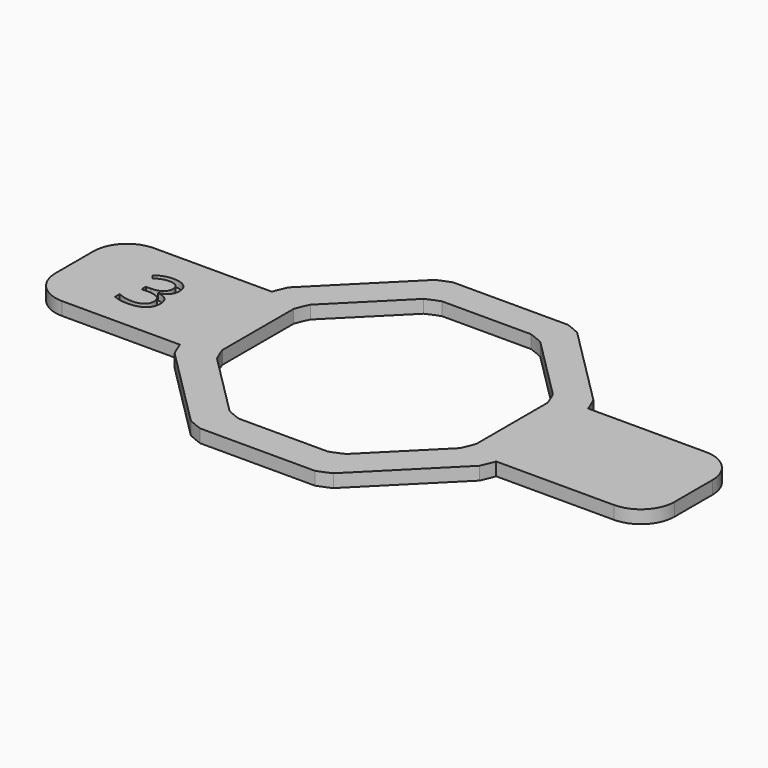
from build123d import *

# Parameters (mm, degrees)
F1_DEPTH     = 1.27
F2_DEPTH     = 1.27
F0_TEXT_SIZE = 7.2862855935
F3_DEPTH     = 0.635


# Not quite as in the source:
# - Text() gives the source's letters only with a copy of the font that has no kerning and outlines rounded to 1/6400 em; it was checked with that copy


with BuildPart() as f1:
    # F0 (on Top) → F1 (new body)
    with BuildSketch(Plane.XY):
        with BuildLine():
            Line((-6.9140659899, 14.7924959485), (-14.7924959485, 6.9140659899))
            ThreePointArc((-14.7924959485, 6.9140659899), (-15.085632938, 6.2486737599), (-15.3488571429, 5.5708912488))
            Line((-15.3488571429, 5.5708912488), (-15.3488571429, -5.5708912488))
            ThreePointArc((-15.3488571429, -5.5708912488), (-15.085632938, -6.2486737599), (-14.7924959485, -6.9140659899))
            Line((-14.7924959485, -6.9140659899), (-6.9140659899, -14.7924959485))
            ThreePointArc((-6.9140659899, -14.7924959485), (-6.2486737599, -15.085632938), (-5.5708912488, -15.3488571429))
            Line((-5.5708912488, -15.3488571429), (5.5708912488, -15.3488571429))
            ThreePointArc((5.5708912488, -15.3488571429), (6.2486737599, -15.085632938), (6.9140659899, -14.7924959485))
            Line((6.9140659899, -14.7924959485), (14.7924959485, -6.9140659899))
            ThreePointArc((14.7924959485, -6.9140659899), (15.085632938, -6.2486737599), (15.3488571429, -5.5708912488))
            Line((15.3488571429, -5.5708912488), (15.3488571429, 5.5708912488))
            ThreePointArc((15.3488571429, 5.5708912488), (15.085632938, 6.2486737599), (14.7924959485, 6.9140659899))
            Line((14.7924959485, 6.9140659899), (6.9140659899, 14.7924959485))
            ThreePointArc((6.9140659899, 14.7924959485), (6.2486737599, 15.085632938), (5.5708912488, 15.3488571429))
            Line((5.5708912488, 15.3488571429), (-5.5708912488, 15.3488571429))
            ThreePointArc((-5.5708912488, 15.3488571429), (-6.2486737599, 15.085632938), (-6.9140659899, 14.7924959485))
        make_face()
        with BuildLine():
            ThreePointArc((11.8104123626, 5.726089617), (12.1074053598, 5.0620161659), (12.366970438, 4.3824395631))
            Line((12.366970438, 4.3824395631), (12.366970438, -4.2562852471))
            ThreePointArc((12.366970438, -4.2562852471), (12.1074053598, -4.9358618499), (11.8104123626, -5.599935301))
            Line((11.8104123626, -5.599935301), (5.7019114684, -11.7084361952))
            ThreePointArc((5.7019114684, -11.7084361952), (5.0378380173, -12.0054291924), (4.3582614145, -12.2649942706))
            Line((4.3582614145, -12.2649942706), (-4.2804633957, -12.2649942706))
            ThreePointArc((-4.2804633957, -12.2649942706), (-4.9600399985, -12.0054291924), (-5.6241134496, -11.7084361952))
            Line((-5.6241134496, -11.7084361952), (-11.7326143438, -5.599935301))
            ThreePointArc((-11.7326143438, -5.599935301), (-12.029607341, -4.9358618499), (-12.2891724192, -4.2562852471))
            Line((-12.2891724192, -4.2562852471), (-12.2891724192, 4.3824395631))
            ThreePointArc((-12.2891724192, 4.3824395631), (-12.029607341, 5.0620161659), (-11.7326143438, 5.726089617))
            Line((-11.7326143438, 5.726089617), (-5.6241134496, 11.8345905111))
            ThreePointArc((-5.6241134496, 11.8345905111), (-4.9600399985, 12.1315835084), (-4.2804633957, 12.3911485866))
            Line((-4.2804633957, 12.3911485866), (4.3582614145, 12.3911485866))
            ThreePointArc((4.3582614145, 12.3911485866), (5.0378380173, 12.1315835084), (5.7019114684, 11.8345905111))
            Line((5.7019114684, 11.8345905111), (11.8104123626, 5.726089617))
        make_face(mode=Mode.SUBTRACT)
    extrude(amount=F1_DEPTH)

    # F0 (on Top) → F2 (join)
    with BuildSketch(Plane.XY):
        with BuildLine():
            Line((-15.3488571429, -5.5708912488), (-15.3488571429, 5.5708912488))
            Line((-15.3488571429, 5.5708912488), (-26.7788571429, 5.5708912488))
            ThreePointArc((-26.7788571429, 5.5708912488), (-29.0880658597, 4.6143856799), (-30.0445714286, 2.3051769631))
            Line((-30.0445714286, 2.3051769631), (-30.0445714286, -2.3051769631))
            ThreePointArc((-30.0445714286, -2.3051769631), (-29.0880658597, -4.6143856799), (-26.7788571429, -5.5708912488))
            Line((-26.7788571429, -5.5708912488), (-15.3488571429, -5.5708912488))
        make_face()
        with BuildLine():
            add(Edge.make_bspline(
                [(-21.2788977233, 2.223162781), (-20.8587978195, 1.8764949743), (-20.8587978195, 1.2719609664)],
                knots=[0, 0, 0, 1, 1, 1], degree=2))
            add(Edge.make_bspline(
                [(-20.8587978195, 1.2719609664), (-20.8587978195, 0.7733057961), (-21.138295181, 0.4568077657)],
                knots=[0, 0, 0, 1, 1, 1], degree=2))
            add(Edge.make_bspline(
                [(-21.138295181, 0.4568077657), (-21.4177925424, 0.1403097352), (-21.9301094982, 0.0332924155)],
                knots=[0, 0, 0, 1, 1, 1], degree=2))
            Line((-21.9301094982, 0.0332924155), (-21.9301094982, 0.0048303624))
            add(Edge.make_bspline(
                [(-21.9301094982, 0.0048303624), (-21.30394433, -0.072586422), (-21.0016773261, -0.3930691399)],
                knots=[0, 0, 0, 1, 1, 1], degree=2))
            add(Edge.make_bspline(
                [(-21.0016773261, -0.3930691399), (-20.6994103222, -0.7135518578), (-20.6994103222, -1.2326997063)],
                knots=[0, 0, 0, 1, 1, 1], degree=2))
            add(Edge.make_bspline(
                [(-20.6994103222, -1.2326997063), (-20.6994103222, -1.9761285333), (-21.2151427243, -2.3768742409)],
                knots=[0, 0, 0, 1, 1, 1], degree=2))
            add(Edge.make_bspline(
                [(-21.2151427243, -2.3768742409), (-21.7308751265, -2.7776199486), (-22.6803692179, -2.7776199486)],
                knots=[0, 0, 0, 1, 1, 1], degree=2))
            add(Edge.make_bspline(
                [(-22.6803692179, -2.7776199486), (-23.0936382289, -2.7776199486), (-23.4368905893, -2.7150034318)],
                knots=[0, 0, 0, 1, 1, 1], degree=2))
            add(Edge.make_bspline(
                [(-23.4368905893, -2.7150034318), (-23.7801429497, -2.6523869149), (-24.1034718729, -2.496414864)],
                knots=[0, 0, 0, 1, 1, 1], degree=2))
            Line((-24.1034718729, -2.496414864), (-24.1034718729, -1.9340046947))
            add(Edge.make_bspline(
                [(-24.1034718729, -1.9340046947), (-23.7653426821, -2.1013615669), (-23.3828126884, -2.1884554494)],
                knots=[0, 0, 0, 1, 1, 1], degree=2))
            add(Edge.make_bspline(
                [(-23.3828126884, -2.1884554494), (-23.0002826947, -2.2755493319), (-22.6587380575, -2.2755493319)],
                knots=[0, 0, 0, 1, 1, 1], degree=2))
            add(Edge.make_bspline(
                [(-22.6587380575, -2.2755493319), (-21.3107752227, -2.2755493319), (-21.3107752227, -1.2190379208)],
                knots=[0, 0, 0, 1, 1, 1], degree=2))
            add(Edge.make_bspline(
                [(-21.3107752227, -1.2190379208), (-21.3107752227, -0.2718207937), (-22.7976328767, -0.2718207937)],
                knots=[0, 0, 0, 1, 1, 1], degree=2))
            Line((-22.7976328767, -0.2718207937), (-23.3099498325, -0.2718207937))
            Line((-23.3099498325, -0.2718207937), (-23.3099498325, 0.2359422336))
            Line((-23.3099498325, 0.2359422336), (-22.7908019839, 0.2359422336))
            add(Edge.make_bspline(
                [(-22.7908019839, 0.2359422336), (-22.1828525297, 0.2359422336), (-21.827076866, 0.5046240149)],
                knots=[0, 0, 0, 1, 1, 1], degree=2))
            add(Edge.make_bspline(
                [(-21.827076866, 0.5046240149), (-21.4713012022, 0.7733057961), (-21.4713012022, 1.2503298061)],
                knots=[0, 0, 0, 1, 1, 1], degree=2))
            add(Edge.make_bspline(
                [(-21.4713012022, 1.2503298061), (-21.4713012022, 1.6305828355), (-21.7325828497, 1.8480329212)],
                knots=[0, 0, 0, 1, 1, 1], degree=2))
            add(Edge.make_bspline(
                [(-21.7325828497, 1.8480329212), (-21.9938644971, 2.0654830068), (-22.442426454, 2.0654830068)],
                knots=[0, 0, 0, 1, 1, 1], degree=2))
            add(Edge.make_bspline(
                [(-22.442426454, 2.0654830068), (-22.7839710912, 2.0654830068), (-23.0862380951, 1.9726967137)],
                knots=[0, 0, 0, 1, 1, 1], degree=2))
            add(Edge.make_bspline(
                [(-23.0862380951, 1.9726967137), (-23.388505099, 1.8799104206), (-23.7767275033, 1.6305828355)],
                knots=[0, 0, 0, 1, 1, 1], degree=2))
            Line((-23.7767275033, 1.6305828355), (-24.0750098198, 2.0290515789))
            add(Edge.make_bspline(
                [(-24.0750098198, 2.0290515789), (-23.7550963429, 2.2817946104), (-23.3372734034, 2.4258125991)],
                knots=[0, 0, 0, 1, 1, 1], degree=2))
            add(Edge.make_bspline(
                [(-23.3372734034, 2.4258125991), (-22.9194504639, 2.5698305878), (-22.4560882395, 2.5698305878)],
                knots=[0, 0, 0, 1, 1, 1], degree=2))
            add(Edge.make_bspline(
                [(-22.4560882395, 2.5698305878), (-21.698997627, 2.5698305878), (-21.2788977233, 2.223162781)],
                knots=[0, 0, 0, 1, 1, 1], degree=2))
        make_face(mode=Mode.SUBTRACT)
        with BuildLine():
            Line((26.7788571429, 5.5708912488), (15.3488571429, 5.5708912488))
            Line((15.3488571429, 5.5708912488), (15.3488571429, -5.5708912488))
            Line((15.3488571429, -5.5708912488), (26.7788571429, -5.5708912488))
            ThreePointArc((26.7788571429, -5.5708912488), (29.0880658597, -4.6143856799), (30.0445714286, -2.3051769631))
            Line((30.0445714286, -2.3051769631), (30.0445714286, 2.3051769631))
            ThreePointArc((30.0445714286, 2.3051769631), (29.0880658597, 4.6143856799), (26.7788571429, 5.5708912488))
        make_face()
    extrude(amount=F2_DEPTH)

    # F0 (on Top) → F3 (join)
    with BuildSketch(Plane.XY):
        with Locations((-24.4381856173, -2.7058955748)):
            Text('3', F0_TEXT_SIZE, font='Open Sans', text_align=(TextAlign.LEFT, TextAlign.BOTTOM))
    extrude(amount=F3_DEPTH)


solid = f1.part
